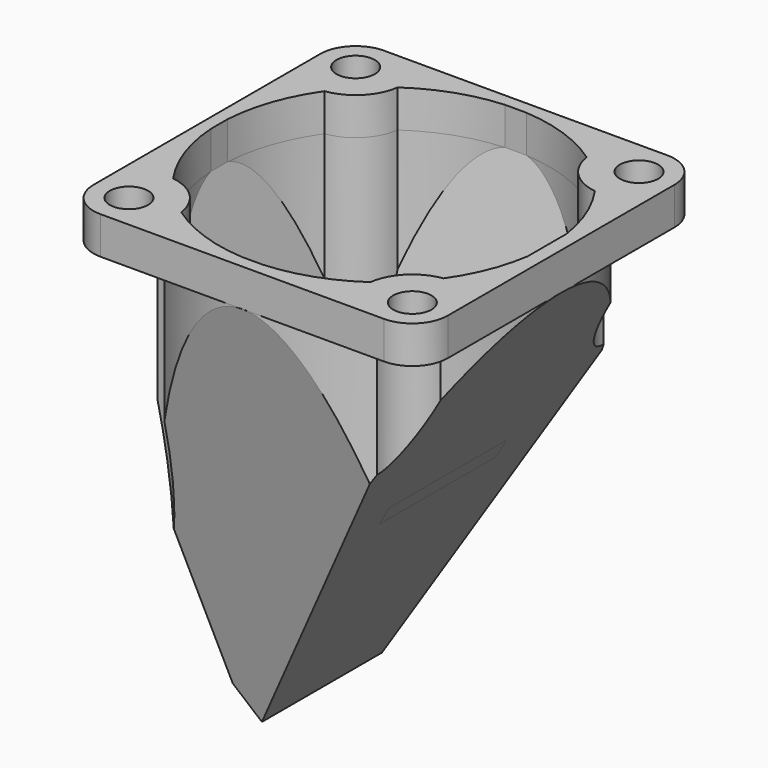
from build123d import *

# Parameters (mm, degrees)
F0_R          = 15
F1_DEPTH      = 50.8
F3_DEPTH      = 50.8
F5_DEPTH      = 16
F5_DEPTH_BACK = 25.4
F6_R          = 2.999994
F7_DEPTH      = 75
F8_T          = -1.0294366
F9_R          = 1.625
F10_DEPTH     = 3.175
F11_R         = 2.999994
F12_W         = 12.402147986
F12_H         = 1.7178952694
F13_DEPTH     = 1.0294366
F15_REACH     = 37.7778044783
F16_DEPTH     = 1.7178952694


# Not quite as in the source:
# - an extrude ends at something that could not be found from the text; its depth is read off the source's solid


with BuildPart() as f1:
    # F0 (on Top) → F1 (new body)
    with BuildSketch(Plane.XY):
        with Locations((0, 15)):
            Circle(F0_R)
    extrude(amount=-F1_DEPTH)

    # F2 (on Front) → F3 (cut)
    with BuildSketch(Plane.XZ):
        Polygon((-15, 0), (-15, -50.8), (15, -50.8), (15, 0), (-5.2591228073, -36.0019072397), (-7.2556595325, -33.5332099912), align=None)
    extrude(amount=-F3_DEPTH, mode=Mode.SUBTRACT)

    # F4 (on Right) → F5 (cut, two sides)
    with BuildSketch(Plane.YZ) as f5_sk:
        Polygon((30, -36.0019072397), (30, 0), (21.35, -36.0019072397), align=None)
        Polygon((8.65, -36.0019072397), (0, 0), (0, -36.0019072397), align=None)
    extrude(amount=-F5_DEPTH, mode=Mode.SUBTRACT)
    extrude(f5_sk.sketch, amount=F5_DEPTH_BACK, mode=Mode.SUBTRACT)

    # F6 (on face) → F7 (cut, through all)
    with BuildSketch(Plane.XY):
        with Locations((12.000006, 27.000006)):
            Circle(F6_R)
        with Locations((12.000006, 2.999994)):
            Circle(F6_R)
        with Locations((-12.000006, 2.999994)):
            Circle(F6_R)
        with Locations((-12.000006, 27.000006)):
            Circle(F6_R)
    extrude(amount=-F7_DEPTH, mode=Mode.SUBTRACT)

    # F8
    f8_openings = [f1.faces().sort_by_distance(p)[0] for p in [
        (0, 15, 0),
    ]]
    offset(amount=F8_T, openings=f8_openings)

    # F9 (on face) → F10 (join)
    with BuildSketch(Plane.XY):
        with BuildLine():
            Line((1.23e-08, 0), (15, 0))
            Line((15, 0), (15, 15))
            ThreePointArc((15, 15), (14.230247099, 10.2565763946), (11.999991, 5.999988))
            ThreePointArc((11.999991, 5.999988), (9.8786898991, 5.1213101009), (9.000012, 3.000009))
            ThreePointArc((9.000012, 3.000009), (4.7434236112, 0.7697529029), (1.23e-08, 0))
        make_face()
        with Locations((12.000006, 2.999994)):
            Circle(F9_R, mode=Mode.SUBTRACT)
        with BuildLine():
            Line((-15, 0), (1.23e-08, 0))
            ThreePointArc((1.23e-08, 0), (-4.7434235996, 0.769752899), (-9.000012, 3.000009))
            ThreePointArc((-9.000012, 3.000009), (-9.8786898991, 5.1213101009), (-11.999991, 5.999988))
            ThreePointArc((-11.999991, 5.999988), (-14.230247099, 10.2565763946), (-15, 15))
            Line((-15, 15), (-15, 0))
        make_face()
        with Locations((-12.000006, 2.999994)):
            Circle(F9_R, mode=Mode.SUBTRACT)
        with BuildLine():
            ThreePointArc((-9.000012, 3.000009), (-4.7434235996, 0.769752899), (1.23e-08, 0))
            ThreePointArc((1.23e-08, 0), (4.7434236112, 0.7697529029), (9.000012, 3.000009))
            ThreePointArc((9.000012, 3.000009), (9.8786898991, 5.1213101009), (11.999991, 5.999988))
            ThreePointArc((11.999991, 5.999988), (14.230247099, 10.2565763946), (15, 15))
            ThreePointArc((15, 15), (14.230247099, 19.7434236054), (11.999991, 24.000012))
            ThreePointArc((11.999991, 24.000012), (9.8786898991, 24.8786898991), (9.000012, 26.999991))
            ThreePointArc((9.000012, 26.999991), (4.7434236018, 29.2302471002), (-7.6e-09, 30))
            ThreePointArc((-7.6e-09, 30), (-4.743423609, 29.2302470978), (-9.000012, 26.999991))
            ThreePointArc((-9.000012, 26.999991), (-9.8786898991, 24.8786898991), (-11.999991, 24.000012))
            ThreePointArc((-11.999991, 24.000012), (-14.230247099, 19.7434236054), (-15, 15))
            ThreePointArc((-15, 15), (-14.230247099, 10.2565763946), (-11.999991, 5.999988))
            ThreePointArc((-11.999991, 5.999988), (-9.8786898991, 5.1213101009), (-9.000012, 3.000009))
        make_face()
        with BuildLine():
            Line((0.9042769799, 1.0587330254), (-0.9042769799, 1.0587330254))
            ThreePointArc((-0.9042769799, 1.0587330254), (-4.6276702262, 1.8181446681), (-8.0086800871, 3.5528307003))
            ThreePointArc((-8.0086800871, 3.5528307003), (-9.1507682984, 5.8492317016), (-11.4471692997, 6.9913199129))
            ThreePointArc((-11.4471692997, 6.9913199129), (-13.1875845683, 10.3886818623), (-13.9434671073, 14.1303065241))
            Line((-13.9434671073, 14.1303065241), (-13.9434671073, 15.8696934759))
            ThreePointArc((-13.9434671073, 15.8696934759), (-13.1875845683, 19.6113181377), (-11.4471692997, 23.0086800871))
            ThreePointArc((-11.4471692997, 23.0086800871), (-9.1507682984, 24.1507682984), (-8.0086800871, 26.4471692997))
            ThreePointArc((-8.0086800871, 26.4471692997), (-4.6276702262, 28.1818553319), (-0.9042769799, 28.9412669746))
            Line((-0.9042769799, 28.9412669746), (0.9042769799, 28.9412669746))
            ThreePointArc((0.9042769799, 28.9412669746), (4.6276702262, 28.1818553319), (8.0086800871, 26.4471692997))
            ThreePointArc((8.0086800871, 26.4471692997), (9.1507682984, 24.1507682984), (11.4471692997, 23.0086800871))
            ThreePointArc((11.4471692997, 23.0086800871), (12.9790918545, 20.1691214289), (13.8187656408, 17.053864133))
            Line((13.8187656408, 17.053864133), (13.8187656408, 12.946135867))
            ThreePointArc((13.8187656408, 12.946135867), (12.9790918545, 9.8308785711), (11.4471692997, 6.9913199129))
            ThreePointArc((11.4471692997, 6.9913199129), (9.1507682984, 5.8492317016), (8.0086800871, 3.5528307003))
            ThreePointArc((8.0086800871, 3.5528307003), (4.6276702262, 1.8181446681), (0.9042769799, 1.0587330254))
        make_face(mode=Mode.SUBTRACT)
        with BuildLine():
            ThreePointArc((11.999991, 24.000012), (14.230247099, 19.7434236054), (15, 15))
            Line((15, 15), (15, 30))
            Line((15, 30), (-7.6e-09, 30))
            ThreePointArc((-7.6e-09, 30), (4.7434236018, 29.2302471002), (9.000012, 26.999991))
            ThreePointArc((9.000012, 26.999991), (9.8786898991, 24.8786898991), (11.999991, 24.000012))
        make_face()
        with Locations((12.000006, 27.000006)):
            Circle(F9_R, mode=Mode.SUBTRACT)
        with BuildLine():
            Line((-15, 30), (-15, 15))
            ThreePointArc((-15, 15), (-14.230247099, 19.7434236054), (-11.999991, 24.000012))
            ThreePointArc((-11.999991, 24.000012), (-9.8786898991, 24.8786898991), (-9.000012, 26.999991))
            ThreePointArc((-9.000012, 26.999991), (-4.743423609, 29.2302470978), (-7.6e-09, 30))
            Line((-7.6e-09, 30), (-15, 30))
        make_face()
        with Locations((-12.000006, 27.000006)):
            Circle(F9_R, mode=Mode.SUBTRACT)
    extrude(amount=F10_DEPTH)

    # F11
    f11_edges = [f1.edges().sort_by_distance(p)[0] for p in [
        (15, 0, 1.5875),
        (-15, 0, 1.5875),
        (-15, 30, 1.5875),
        (15, 30, 1.5875),
    ]]
    fillet(f11_edges, radius=F11_R)

    # F12 (on face) → F13 (cut, through all)
    with BuildSketch(Plane(origin=(11.3924813609, 0, -6.4108181112), x_dir=(0, 1, 0), z_dir=(0.8714922589, 0, -0.4904092603))):
        with Locations((14.4248786382, -12.1594956145)):
            Rectangle(F12_W, F12_H)
    extrude(amount=-F13_DEPTH, mode=Mode.SUBTRACT)

    f15_end = f1.faces().sort_by_distance((-6.2722387902, 15, -34.7491996848))[0]
    # F14 (on face) → F15 (cut, up to a face of the model that its end follows)
    with BuildSketch(Plane(origin=(-6.3843651243, 0, -11.3454725151), x_dir=(0.8714922589, 0, -0.4904092603), z_dir=(0.4904092603, 0, 0.8714922589))):
        Polygon((12.0429472841, 9.2698510415), (12.0429472841, 20.7301489585), (10.7223677877, 20.9956137981), (10.7223677877, 9.0043862019), align=None)
    f15_long = extrude(amount=-F15_REACH, mode=Mode.PRIVATE)
    add(split(f15_long, bisect_by=f15_end, keep=Keep.BOTTOM, mode=Mode.PRIVATE), mode=Mode.SUBTRACT)

    # F16 (add, through all): a face of the model
    f16_faces = [f1.faces().sort_by_distance(p)[0] for p in [
        (4.5595432226, 14.4248786382, -17.5038680055),
    ]]
    extrude(f16_faces, amount=F16_DEPTH)


solid = f1.part
